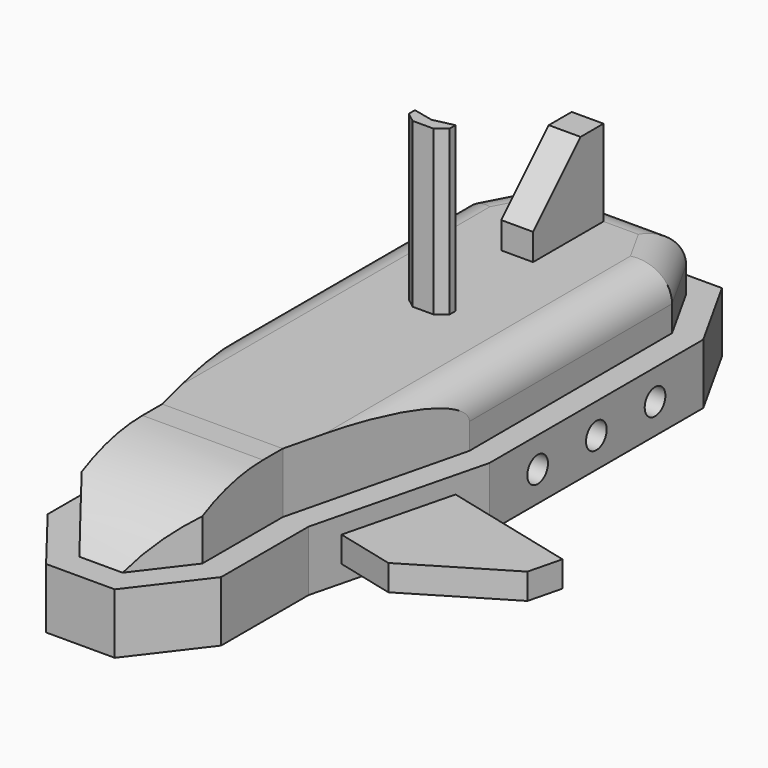
from build123d import *

# Parameters (mm, degrees)
F1_DEPTH    = 8.89
F3_DEPTH    = 8.89
F4_T1_DEPTH = 99.9162053314
F5_DEPTH    = 8.89
F6_R        = 5.08
F8_D        = 3.81
F8_DEPTH    = 3.81
F8_TIP      = 1.1446394792
F10_D       = 3.81
F10_DEPTH   = 3.81
F10_TIP     = 1.1446394792
F11_R       = 1.905
F12_DEPTH   = 3.81
F14_DEPTH   = 38.1
F15_DEPTH   = 38.1
F16_DEPTH   = 38.1
F17_W       = 4.6861195005
F17_H       = 12.987878806
F18_DEPTH   = 12.7
F19_SIZE    = 8.763
F20_W       = 16.51
F20_H       = 3.81
F21_DEPTH   = 20.32
F22_SIZE    = 11.43


# Not quite as in the source:
# - a fillet or chamfer that OpenCascade refuses, or shapes differently, is made with other operations: its cross-section is extruded or revolved along the edge and cut away or added


with BuildPart() as f1:
    # F0 (on Top) → F1 (new body)
    with BuildSketch(Plane.XY):
        Polygon((19.05, 26.7226453871), (12.7, 38.1), (-12.7, 38.1), (-19.05, 26.1296909302), (-19.05, -12.7), (-12.7, -38.1), (-12.7, -54.4537100359), (-5.0853045448, -64.2633512616), (5.0406523641, -64.2633512616), (12.7, -54.2242169015), (12.7, -38.1), (19.05, -12.7), align=None)
    extrude(amount=F1_DEPTH)

    # F2 (on face) → F5 (join)
    with BuildSketch(Plane.XY.offset(8.89)):
        Polygon((-15.24, -12.2309675664), (-8.89, -38.1), (8.89, -38.1), (15.3537570744, -11.7759392686), (15.24, 25.7313851458), (10.4632125856, 34.29), (-10.4082323758, 34.29), (-15.24, 25.1816926275), align=None)
    extrude(amount=F5_DEPTH)

    # F6
    f6_edges = [f1.edges().sort_by_distance(p)[0] for p in [
        (-15.24, 6.475363, 17.78),
        (15.296879, 6.977723, 17.78),
        (-12.824116, 29.735846, 17.78),
        (12.851606, 30.010693, 17.78),
        (0.02749, 34.29, 17.78),
    ]]
    fillet(f6_edges, radius=F6_R)

    # F8
    with Locations(Plane.YZ.offset(19.05)):
        with Locations((-3.81, 4.445), (7.0104, 4.445), (17.8326453871, 4.445)):
            Hole(F8_D / 2, depth=F8_DEPTH)
            with Locations((0, 0, -(F8_DEPTH + F8_TIP / 2))):  # 118° drill point
                Cone(0, F8_D / 2, F8_TIP, mode=Mode.SUBTRACT)

    # F10
    with Locations(Plane(origin=(-19.05, 0, 0), x_dir=(0, -1, 0), z_dir=(-1, 0, 0))):
        with Locations((-17.2396909302, 4.445), (-6.684313026, 4.445), (3.81, 4.445)):
            Hole(F10_D / 2, depth=F10_DEPTH)
            with Locations((0, 0, -(F10_DEPTH + F10_TIP / 2))):  # 118° drill point
                Cone(0, F10_D / 2, F10_TIP, mode=Mode.SUBTRACT)


with BuildPart() as f3:
    # F2 (on face) → F3 (new body)
    with BuildSketch(Plane.XY.offset(8.89)):
        Polygon((8.89, -38.1), (-8.89, -38.1), (-8.89, -52.936759997), (-3.2196400783, -60.4533512616), (-0.0223260903, -60.4533512616), (3.1552241252, -60.4533512616), (8.89, -52.936759997), align=None)
    extrude(amount=F3_DEPTH)

    # F4: fillet of radius 24.13 on 1 edges, made by hand

    # F4_s2 → F4_t1 (cut)
    with BuildSketch(Plane.YZ.offset(-49.9903106423)):
        with BuildLine():
            ThreePointArc((-41.745083036, 17.78), (-52.1016196193, 15.4444729232), (-60.4533512616, 8.89))
            Line((-60.4533512616, 8.89), (-60.4533512616, 17.78))
            Line((-60.4533512616, 17.78), (-41.745083036, 17.78))
        make_face()
    extrude(amount=F4_T1_DEPTH, mode=Mode.SUBTRACT)


with BuildPart() as f12:
    # F11 (on Top) → F12 (new body)
    with BuildSketch(Plane.XY):
        Circle(F11_R)
    extrude(amount=F12_DEPTH)

    # F13 (on face) → F14 (join)
    with BuildSketch(Plane.XY.offset(3.81)):
        with BuildLine():
            Line((0, -1.1266035726), (1.5361606004, -1.1266035726))
            ThreePointArc((1.5361606004, -1.1266035726), (1.8104434462, -0.592722134), (1.905, 0))
            ThreePointArc((1.905, 0), (1.8558119687, 0.4301010776), (1.7107879927, 0.837991315))
            Line((1.7107879927, 0.837991315), (0, 0.4536258639))
            Line((0, 0.4536258639), (-1.7107879927, 0.837991315))
            ThreePointArc((-1.7107879927, 0.837991315), (-1.8975186586, -0.1686651723), (-1.5361606004, -1.1266035726))
            Line((-1.5361606004, -1.1266035726), (0, -1.1266035726))
        make_face()
    extrude(amount=F14_DEPTH)

    # F13 (on face) → F15 (join)
    with BuildSketch(Plane.XY.offset(3.81)):
        with BuildLine():
            Line((-2.9953841586, 0), (-1.5361606004, -1.1266035726))
            ThreePointArc((-1.5361606004, -1.1266035726), (-1.8975186586, -0.1686651723), (-1.7107879927, 0.837991315))
            Line((-1.7107879927, 0.837991315), (-2.9953841586, 1.1266035726))
            Line((-2.9953841586, 1.1266035726), (-2.9953841586, 0))
        make_face()
    extrude(amount=F15_DEPTH)

    # F13 (on face) → F16 (join)
    with BuildSketch(Plane.XY.offset(3.81)):
        with BuildLine():
            ThreePointArc((1.905, 0), (1.8104434462, -0.592722134), (1.5361606004, -1.1266035726))
            Line((1.5361606004, -1.1266035726), (2.9953841586, 0))
            Line((2.9953841586, 0), (2.9953841586, 1.1266035726))
            Line((2.9953841586, 1.1266035726), (1.7107879927, 0.837991315))
            ThreePointArc((1.7107879927, 0.837991315), (1.8558119687, 0.4301010776), (1.905, 0))
        make_face()
    extrude(amount=F16_DEPTH)


with BuildPart() as f18:
    # F17 (on face) → F18 (new body)
    with BuildSketch(Plane.XY.offset(17.78)):
        with Locations((0, 22.716060597)):
            Rectangle(F17_W, F17_H)
    extrude(amount=F18_DEPTH)

    # F19
    f19_edges = [f18.edges().sort_by_distance(p)[0] for p in [
        (0, 16.222121, 30.48),
    ]]
    chamfer(f19_edges, length=F19_SIZE)


with BuildPart() as f21:
    # F20 (on face) → F21 (new body)
    with BuildSketch(Plane(origin=(20.9176470588, -5.2294117647, 0), x_dir=(0.242535625, 0.9701425001, 0), z_dir=(0.9701425001, -0.242535625, 0))):
        with Locations((-20.8566915244, 4.445)):
            Rectangle(F20_W, F20_H)
    extrude(amount=F21_DEPTH)

    # F22
    f22_edges = [f21.edges().sort_by_distance(p)[0] for p in [
        (33.57032, -38.400225, 4.445),
    ]]
    chamfer(f22_edges, length=F22_SIZE)


solid = Compound([f1.part, f3.part, f12.part, f18.part, f21.part])
